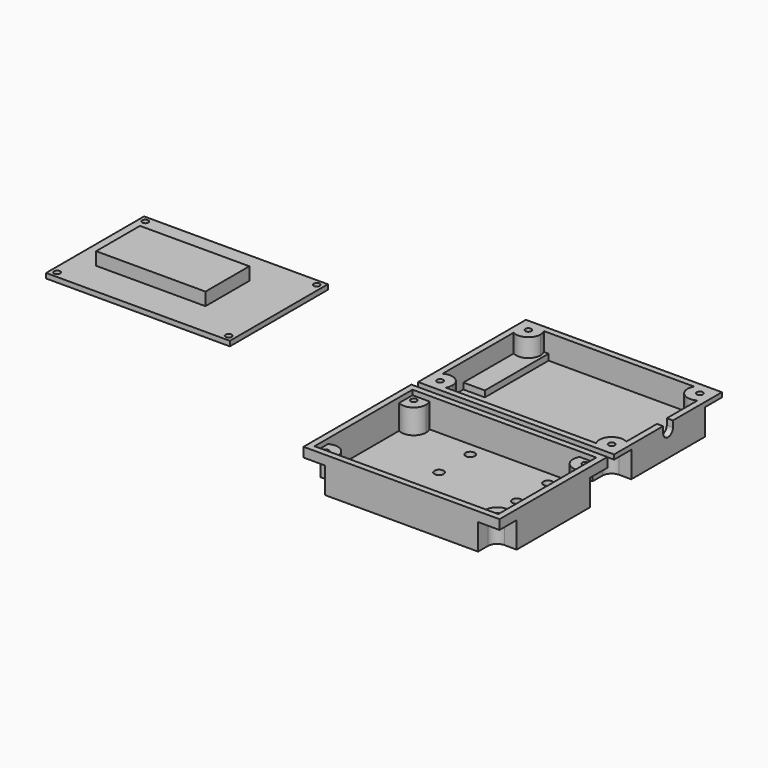
from build123d import *

# Parameters (mm, degrees)
F0_W      = 60
F0_H      = 40
F0_R      = 1
F1_DEPTH  = 1.6
F3_W      = 35.7
F3_H      = 17.9
F4_DEPTH  = 4.2
F5_W      = 64
F5_H      = 44
F5_R      = 1
F6_DEPTH  = 2
F7_R      = 1
F8_DEPTH  = 8
F9_W      = 64
F9_H      = 44
F9_R      = 1
F10_DEPTH = 2
F11_R     = 1
F12_DEPTH = 8
F13_W     = 64
F13_H     = 44
F13_W_2   = 60
F13_H_2   = 40
F14_DEPTH = 1.6
F16_DEPTH = 8.5
F18_DEPTH = 8.5
F20_DEPTH = 25.4
F21_R     = 1.5
F22_DEPTH = 25.4
F23_W     = 9
F23_H     = 28
F24_DEPTH = 4
F25_W     = 7
F25_H     = 26
F26_DEPTH = 2
F27_R     = 1
F28_DEPTH = 25.4


with BuildPart() as f1:
    # F0 (on Top) → F1 (new body)
    with BuildSketch(Plane.XY):
        with Locations((-71.7097583413, 11.8171558529)):
            Rectangle(F0_W, F0_H)
        with Locations((-99.7097583413, -6.1828441471)):
            Circle(F0_R, mode=Mode.SUBTRACT)
        with Locations((-43.7097583413, -6.1828441471)):
            Circle(F0_R, mode=Mode.SUBTRACT)
        with Locations((-99.7097583413, 29.8171558529)):
            Circle(F0_R, mode=Mode.SUBTRACT)
        with Locations((-43.7097583413, 29.8171558529)):
            Circle(F0_R, mode=Mode.SUBTRACT)
    extrude(amount=F1_DEPTH)

    # F3 (on face) → F4 (join)
    with BuildSketch(Plane.XY.offset(1.6)):
        with Locations((-76.3597583413, 11.8171558529)):
            Rectangle(F3_W, F3_H)
    extrude(amount=F4_DEPTH)


with BuildPart() as f6:
    # F5 (on Top) → F6 (new body)
    with BuildSketch(Plane.XY):
        with Locations((52.0504697859, 13.4392828941)):
            Rectangle(F5_W, F5_H)
        with Locations((24.0504697859, -4.5607171059)):
            Circle(F5_R, mode=Mode.SUBTRACT)
        with Locations((80.0504697859, -4.5607171059)):
            Circle(F5_R, mode=Mode.SUBTRACT)
        with Locations((24.0504697859, 31.4392828941)):
            Circle(F5_R, mode=Mode.SUBTRACT)
        with Locations((80.0504697859, 31.4392828941)):
            Circle(F5_R, mode=Mode.SUBTRACT)
    extrude(amount=F6_DEPTH)

    # F7 (on face) → F8 (join)
    with BuildSketch(Plane.XY.offset(2)):
        with BuildLine():
            Line((22.0504697859, 33.4392828941), (27.5145714011, 33.4392828941))
            ThreePointArc((27.5145714011, 33.4392828941), (26.0504697859, 34.9033845093), (24.0504697859, 35.4392828941))
            ThreePointArc((24.0504697859, 35.4392828941), (21.2220426612, 34.2677100189), (20.0504697859, 31.4392828941))
            ThreePointArc((20.0504697859, 31.4392828941), (20.5863681708, 29.4392828941), (22.0504697859, 27.975181279))
            Line((22.0504697859, 27.975181279), (22.0504697859, 33.4392828941))
        make_face()
        with BuildLine():
            ThreePointArc((24.0504697859, 35.4392828941), (26.0504697859, 34.9033845093), (27.5145714011, 33.4392828941))
            Line((27.5145714011, 33.4392828941), (76.5863681708, 33.4392828941))
            ThreePointArc((76.5863681708, 33.4392828941), (78.0504697859, 34.9033845093), (80.0504697859, 35.4392828941))
            Line((80.0504697859, 35.4392828941), (24.0504697859, 35.4392828941))
        make_face()
        with BuildLine():
            Line((22.0504697859, -1.0966154907), (22.0504697859, 27.975181279))
            ThreePointArc((22.0504697859, 27.975181279), (20.5863681708, 29.4392828941), (20.0504697859, 31.4392828941))
            Line((20.0504697859, 31.4392828941), (20.0504697859, -4.5607170954))
            ThreePointArc((20.0504697859, -4.5607170954), (20.5863681734, -2.5607171013), (22.0504697859, -1.0966154907))
        make_face()
        with BuildLine():
            ThreePointArc((20.0504697859, 31.4392828941), (21.2220426612, 34.2677100189), (24.0504697859, 35.4392828941))
            Line((24.0504697859, 35.4392828941), (20.0504697859, 35.4392828941))
            Line((20.0504697859, 35.4392828941), (20.0504697859, 31.4392828941))
        make_face()
        with BuildLine():
            ThreePointArc((80.0504697859, 35.4392828941), (78.0504697859, 34.9033845093), (76.5863681708, 33.4392828941))
            Line((76.5863681708, 33.4392828941), (82.0504697859, 33.4392828941))
            Line((82.0504697859, 33.4392828941), (82.0504697859, 27.975181279))
            ThreePointArc((82.0504697859, 27.975181279), (83.5145714011, 29.4392828941), (84.0504697859, 31.4392828941))
            ThreePointArc((84.0504697859, 31.4392828941), (82.8788969107, 34.2677100189), (80.0504697859, 35.4392828941))
        make_face()
        with BuildLine():
            Line((22.0504697859, -6.5607171059), (22.0504697859, -1.0966154907))
            ThreePointArc((22.0504697859, -1.0966154907), (20.5863681734, -2.5607171013), (20.0504697859, -4.5607170954))
            ThreePointArc((20.0504697859, -4.5607170954), (21.2220426575, -7.3891442269), (24.0504697859, -8.5607171059))
            ThreePointArc((24.0504697859, -8.5607171059), (26.0504697859, -8.024818721), (27.5145714011, -6.5607171059))
            Line((27.5145714011, -6.5607171059), (22.0504697859, -6.5607171059))
        make_face()
        with BuildLine():
            Line((84.0504697859, 35.4392828941), (80.0504697859, 35.4392828941))
            ThreePointArc((80.0504697859, 35.4392828941), (82.8788969107, 34.2677100189), (84.0504697859, 31.4392828941))
            Line((84.0504697859, 31.4392828941), (84.0504697859, 35.4392828941))
        make_face()
        with BuildLine():
            ThreePointArc((84.0504697859, 31.4392828941), (83.5145714011, 29.4392828941), (82.0504697859, 27.975181279))
            Line((82.0504697859, 27.975181279), (82.0504697859, -1.0966154907))
            ThreePointArc((82.0504697859, -1.0966154907), (83.5145714011, -2.5607171059), (84.0504697859, -4.5607171059))
            Line((84.0504697859, -4.5607171059), (84.0504697859, 31.4392828941))
        make_face()
        with BuildLine():
            ThreePointArc((24.0504697859, -8.5607171059), (21.2220426575, -7.3891442269), (20.0504697859, -4.5607170954))
            Line((20.0504697859, -4.5607170954), (20.0504697859, -8.5607171059))
            Line((20.0504697859, -8.5607171059), (24.0504697859, -8.5607171059))
        make_face()
        with BuildLine():
            ThreePointArc((84.0504697859, -4.5607171059), (83.5145714011, -2.5607171059), (82.0504697859, -1.0966154907))
            Line((82.0504697859, -1.0966154907), (82.0504697859, -6.5607171059))
            Line((82.0504697859, -6.5607171059), (76.5863681708, -6.5607171059))
            ThreePointArc((76.5863681708, -6.5607171059), (78.0504697859, -8.024818721), (80.0504697859, -8.5607171059))
            ThreePointArc((80.0504697859, -8.5607171059), (82.8788969107, -7.3891442306), (84.0504697859, -4.5607171059))
        make_face()
        with BuildLine():
            ThreePointArc((27.5145714011, -6.5607171059), (26.0504697859, -8.024818721), (24.0504697859, -8.5607171059))
            Line((24.0504697859, -8.5607171059), (80.0504697859, -8.5607171059))
            ThreePointArc((80.0504697859, -8.5607171059), (78.0504697859, -8.024818721), (76.5863681708, -6.5607171059))
            Line((76.5863681708, -6.5607171059), (27.5145714011, -6.5607171059))
        make_face()
        with BuildLine():
            Line((84.0504697859, -8.5607171059), (84.0504697859, -4.5607171059))
            ThreePointArc((84.0504697859, -4.5607171059), (82.8788969107, -7.3891442306), (80.0504697859, -8.5607171059))
            Line((80.0504697859, -8.5607171059), (84.0504697859, -8.5607171059))
        make_face()
        with BuildLine():
            ThreePointArc((22.0504697859, 27.975181279), (26.0504697859, 27.975181279), (28.0504697859, 31.4392828941))
            ThreePointArc((28.0504697859, 31.4392828941), (27.9141730911, 32.4745590745), (27.5145714011, 33.4392828941))
            Line((27.5145714011, 33.4392828941), (22.0504697859, 33.4392828941))
            Line((22.0504697859, 33.4392828941), (22.0504697859, 27.975181279))
        make_face()
        with Locations((24.0504697859, 31.4392828941)):
            Circle(F7_R, mode=Mode.SUBTRACT)
        with BuildLine():
            ThreePointArc((28.0504697859, -4.5607171059), (26.0504697859, -1.0966154907), (22.0504697859, -1.0966154907))
            Line((22.0504697859, -1.0966154907), (22.0504697859, -6.5607171059))
            Line((22.0504697859, -6.5607171059), (27.5145714011, -6.5607171059))
            ThreePointArc((27.5145714011, -6.5607171059), (27.9141730911, -5.5959932863), (28.0504697859, -4.5607171059))
        make_face()
        with Locations((24.0504697859, -4.5607171059)):
            Circle(F7_R, mode=Mode.SUBTRACT)
        with BuildLine():
            Line((82.0504697859, -6.5607171059), (82.0504697859, -1.0966154907))
            ThreePointArc((82.0504697859, -1.0966154907), (77.2220426612, -1.7322899811), (76.5863681708, -6.5607171059))
            Line((76.5863681708, -6.5607171059), (82.0504697859, -6.5607171059))
        make_face()
        with Locations((80.0504697859, -4.5607171059)):
            Circle(F7_R, mode=Mode.SUBTRACT)
        with BuildLine():
            Line((82.0504697859, 33.4392828941), (76.5863681708, 33.4392828941))
            ThreePointArc((76.5863681708, 33.4392828941), (77.2220426612, 28.6108557694), (82.0504697859, 27.975181279))
            Line((82.0504697859, 27.975181279), (82.0504697859, 33.4392828941))
        make_face()
        with Locations((80.0504697859, 31.4392828941)):
            Circle(F7_R, mode=Mode.SUBTRACT)
    extrude(amount=F8_DEPTH)

    # F17 (on face) → F18 (cut)
    with BuildSketch(Plane(origin=(0, 0, 0), x_dir=(1, 0, 0), z_dir=(0, 0, -1))):
        with BuildLine():
            ThreePointArc((80.0504697859, 1.5607171059), (82.1717901295, 2.4393967623), (83.0504697859, 4.5607171059))
            ThreePointArc((83.0504697859, 4.5607171059), (80.0504697859, 7.5607171059), (77.0504697859, 4.5607171059))
            ThreePointArc((77.0504697859, 4.5607171059), (77.9291494424, 2.4393967623), (80.0504697859, 1.5607171059))
        make_face()
        with BuildLine():
            ThreePointArc((77.0504697859, -31.4392828941), (80.0504697859, -34.4392828941), (83.0504697859, -31.4392828941))
            ThreePointArc((83.0504697859, -31.4392828941), (82.1717901295, -29.3179625506), (80.0504697859, -28.4392828941))
            ThreePointArc((80.0504697859, -28.4392828941), (77.9291494424, -29.3179625506), (77.0504697859, -31.4392828941))
        make_face()
        with BuildLine():
            ThreePointArc((24.0504697859, 1.5607171059), (26.1717901295, 2.4393967623), (27.0504697859, 4.5607171059))
            ThreePointArc((27.0504697859, 4.5607171059), (21.9291494424, 6.6820374494), (24.0504697859, 1.5607171059))
        make_face()
        with BuildLine():
            ThreePointArc((24.0504697859, -28.4392828941), (21.9291494424, -33.5606032377), (27.0504697859, -31.4392828941))
            ThreePointArc((27.0504697859, -31.4392828941), (26.1717901295, -29.3179625506), (24.0504697859, -28.4392828941))
        make_face()
        with BuildLine():
            ThreePointArc((77.0504697859, 4.5607171059), (80.0504697859, 7.5607171059), (83.0504697859, 4.5607171059))
            ThreePointArc((83.0504697859, 4.5607171059), (82.1717901295, 2.4393967623), (80.0504697859, 1.5607171059))
            Line((80.0504697859, 1.5607171059), (84.0504697859, 1.5607171059))
            Line((84.0504697859, 1.5607171059), (84.0504697859, 8.5607171059))
            Line((84.0504697859, 8.5607171059), (77.0504697859, 8.5607171059))
            Line((77.0504697859, 8.5607171059), (77.0504697859, 4.5607171059))
        make_face()
        with BuildLine():
            Line((84.0504697859, -35.4392828941), (84.0504697859, -28.4392828941))
            Line((84.0504697859, -28.4392828941), (80.0504697859, -28.4392828941))
            ThreePointArc((80.0504697859, -28.4392828941), (82.1717901295, -29.3179625506), (83.0504697859, -31.4392828941))
            ThreePointArc((83.0504697859, -31.4392828941), (80.0504697859, -34.4392828941), (77.0504697859, -31.4392828941))
            Line((77.0504697859, -31.4392828941), (77.0504697859, -35.4392828941))
            Line((77.0504697859, -35.4392828941), (84.0504697859, -35.4392828941))
        make_face()
        with BuildLine():
            Line((27.0504697859, 4.5607171059), (27.0504697859, 8.5607171059))
            Line((27.0504697859, 8.5607171059), (20.0504697859, 8.5607171059))
            Line((20.0504697859, 8.5607171059), (20.0504697859, 1.5607171059))
            Line((20.0504697859, 1.5607171059), (24.0504697859, 1.5607171059))
            ThreePointArc((24.0504697859, 1.5607171059), (21.9291494424, 6.6820374494), (27.0504697859, 4.5607171059))
        make_face()
        with BuildLine():
            Line((24.0504697859, -28.4392828941), (20.0504697859, -28.4392828941))
            Line((20.0504697859, -28.4392828941), (20.0504697859, -35.4392828941))
            Line((20.0504697859, -35.4392828941), (27.0504697859, -35.4392828941))
            Line((27.0504697859, -35.4392828941), (27.0504697859, -31.4392828941))
            ThreePointArc((27.0504697859, -31.4392828941), (21.9291494424, -33.5606032377), (24.0504697859, -28.4392828941))
        make_face()
    extrude(amount=-F18_DEPTH, mode=Mode.SUBTRACT)

    # F19 (on face) → F20 (cut)
    with BuildSketch(Plane.YZ.offset(84.0504697859)):
        with BuildLine():
            ThreePointArc((13.4392828941, 10), (12.0250693318, 9.4142135624), (11.4392828941, 8))
            ThreePointArc((11.4392828941, 8), (13.4392828941, 6), (15.4392828941, 8))
            ThreePointArc((15.4392828941, 8), (14.8534964565, 9.4142135624), (13.4392828941, 10))
        make_face()
        with BuildLine():
            ThreePointArc((13.4392828941, 10), (14.8534964565, 9.4142135624), (15.4392828941, 8))
            Line((15.4392828941, 8), (15.4392828941, 10))
            Line((15.4392828941, 10), (13.4392828941, 10))
        make_face()
        with BuildLine():
            Line((11.4392828941, 10), (11.4392828941, 8))
            ThreePointArc((11.4392828941, 8), (12.0250693318, 9.4142135624), (13.4392828941, 10))
            Line((13.4392828941, 10), (11.4392828941, 10))
        make_face()
    extrude(amount=-F20_DEPTH, mode=Mode.SUBTRACT)

    # F23 (on face) → F24 (join)
    with BuildSketch(Plane(origin=(0, 0, 0), x_dir=(1, 0, 0), z_dir=(0, 0, -1))):
        with Locations((24.5504697859, -21.4392828941)):
            Rectangle(F23_W, F23_H)
    extrude(amount=-F24_DEPTH)

    # F25 (on face) → F26 (cut)
    with BuildSketch(Plane(origin=(0, 0, 0), x_dir=(1, 0, 0), z_dir=(0, 0, -1))):
        with Locations((23.5504697859, -22.4392828941)):
            Rectangle(F25_W, F25_H)
    extrude(amount=-F26_DEPTH, mode=Mode.SUBTRACT)

    # F27 (on face) → F28 (cut)
    with BuildSketch(Plane(origin=(0, 0, 8.5), x_dir=(1, 0, 0), z_dir=(0, 0, -1))):
        with BuildLine():
            ThreePointArc((24.0504697859, -28.4392828941), (21.9291494424, -33.5606032377), (27.0504697859, -31.4392828941))
            ThreePointArc((27.0504697859, -31.4392828941), (26.1717901295, -29.3179625506), (24.0504697859, -28.4392828941))
        make_face()
        with Locations((24.0504697859, -31.4392828941)):
            Circle(F27_R, mode=Mode.SUBTRACT)
        with BuildLine():
            Line((20.0504697859, -28.4392828941), (20.0504697859, -35.4392828941))
            Line((20.0504697859, -35.4392828941), (27.0504697859, -35.4392828941))
            Line((27.0504697859, -35.4392828941), (27.0504697859, -31.4392828941))
            ThreePointArc((27.0504697859, -31.4392828941), (21.9291494424, -33.5606032377), (24.0504697859, -28.4392828941))
            Line((24.0504697859, -28.4392828941), (20.0504697859, -28.4392828941))
        make_face()
        with Locations((24.0504697859, -31.4392828941)):
            Circle(F27_R)
    extrude(amount=F28_DEPTH, mode=Mode.SUBTRACT)


with BuildPart() as f10:
    # F9 (on Top) → F10 (new body)
    with BuildSketch(Plane.XY):
        with Locations((53.5033790469, -35.1341663599)):
            Rectangle(F9_W, F9_H)
        with Locations((25.5033790469, -53.1341663599)):
            Circle(F9_R, mode=Mode.SUBTRACT)
        with Locations((81.5033790469, -53.1341663599)):
            Circle(F9_R, mode=Mode.SUBTRACT)
        with Locations((25.5033790469, -17.1341663599)):
            Circle(F9_R, mode=Mode.SUBTRACT)
        with Locations((81.5033790469, -17.1341663599)):
            Circle(F9_R, mode=Mode.SUBTRACT)
    extrude(amount=F10_DEPTH)

    # F11 (on face) → F12 (join)
    with BuildSketch(Plane.XY.offset(2)):
        with BuildLine():
            Line((23.5033790469, -15.1341663599), (28.9674806621, -15.1341663599))
            ThreePointArc((28.9674806621, -15.1341663599), (27.5033790469, -13.6700647448), (25.5033790469, -13.1341663599))
            ThreePointArc((25.5033790469, -13.1341663599), (22.6749519222, -14.3057392352), (21.5033790469, -17.1341663599))
            ThreePointArc((21.5033790469, -17.1341663599), (22.0392774318, -19.1341663599), (23.5033790469, -20.598267975))
            Line((23.5033790469, -20.598267975), (23.5033790469, -15.1341663599))
        make_face()
        with BuildLine():
            ThreePointArc((25.5033790469, -13.1341663599), (27.5033790469, -13.6700647448), (28.9674806621, -15.1341663599))
            Line((28.9674806621, -15.1341663599), (78.0392774318, -15.1341663599))
            ThreePointArc((78.0392774318, -15.1341663599), (79.5033790396, -13.670064749), (81.50337903, -13.1341663599))
            Line((81.50337903, -13.1341663599), (25.5033790469, -13.1341663599))
        make_face()
        with BuildLine():
            Line((23.5033790469, -49.6700647448), (23.5033790469, -20.598267975))
            ThreePointArc((23.5033790469, -20.598267975), (22.0392774318, -19.1341663599), (21.5033790469, -17.1341663599))
            Line((21.5033790469, -17.1341663599), (21.5033790469, -53.1341663599))
            ThreePointArc((21.5033790469, -53.1341663599), (22.0392774318, -51.1341663599), (23.5033790469, -49.6700647448))
        make_face()
        with BuildLine():
            ThreePointArc((21.5033790469, -17.1341663599), (22.6749519222, -14.3057392352), (25.5033790469, -13.1341663599))
            Line((25.5033790469, -13.1341663599), (21.5033790469, -13.1341663599))
            Line((21.5033790469, -13.1341663599), (21.5033790469, -17.1341663599))
        make_face()
        with BuildLine():
            ThreePointArc((81.50337903, -13.1341663599), (79.5033790396, -13.670064749), (78.0392774318, -15.1341663599))
            Line((78.0392774318, -15.1341663599), (83.5033790469, -15.1341663599))
            Line((83.5033790469, -15.1341663599), (83.5033790469, -20.598267975))
            ThreePointArc((83.5033790469, -20.598267975), (84.9674806621, -19.1341663599), (85.5033790469, -17.1341663599))
            ThreePointArc((85.5033790469, -17.1341663599), (84.3318061657, -14.3057392292), (81.50337903, -13.1341663599))
        make_face()
        with BuildLine():
            Line((23.5033790469, -55.1341663599), (23.5033790469, -49.6700647448))
            ThreePointArc((23.5033790469, -49.6700647448), (22.0392774318, -51.1341663599), (21.5033790469, -53.1341663599))
            ThreePointArc((21.5033790469, -53.1341663599), (22.6749519222, -55.9625934846), (25.5033790469, -57.1341663599))
            ThreePointArc((25.5033790469, -57.1341663599), (27.5033790469, -56.598267975), (28.9674806621, -55.1341663599))
            Line((28.9674806621, -55.1341663599), (23.5033790469, -55.1341663599))
        make_face()
        with BuildLine():
            Line((85.5033790469, -13.1341663599), (81.50337903, -13.1341663599))
            ThreePointArc((81.50337903, -13.1341663599), (84.3318061657, -14.3057392292), (85.5033790469, -17.1341663599))
            Line((85.5033790469, -17.1341663599), (85.5033790469, -13.1341663599))
        make_face()
        with BuildLine():
            ThreePointArc((85.5033790469, -17.1341663599), (84.9674806621, -19.1341663599), (83.5033790469, -20.598267975))
            Line((83.5033790469, -20.598267975), (83.5033790469, -49.6700647448))
            ThreePointArc((83.5033790469, -49.6700647448), (84.9674806621, -51.1341663599), (85.5033790469, -53.1341663599))
            Line((85.5033790469, -53.1341663599), (85.5033790469, -17.1341663599))
        make_face()
        with BuildLine():
            ThreePointArc((25.5033790469, -57.1341663599), (22.6749519222, -55.9625934846), (21.5033790469, -53.1341663599))
            Line((21.5033790469, -53.1341663599), (21.5033790469, -57.1341663599))
            Line((21.5033790469, -57.1341663599), (25.5033790469, -57.1341663599))
        make_face()
        with BuildLine():
            ThreePointArc((85.5033790469, -53.1341663599), (84.9674806621, -51.1341663599), (83.5033790469, -49.6700647448))
            Line((83.5033790469, -49.6700647448), (83.5033790469, -55.1341663599))
            Line((83.5033790469, -55.1341663599), (78.0392774318, -55.1341663599))
            ThreePointArc((78.0392774318, -55.1341663599), (79.5033790469, -56.598267975), (81.5033790469, -57.1341663599))
            ThreePointArc((81.5033790469, -57.1341663599), (84.3318061717, -55.9625934846), (85.5033790469, -53.1341663599))
        make_face()
        with BuildLine():
            ThreePointArc((28.9674806621, -55.1341663599), (27.5033790469, -56.598267975), (25.5033790469, -57.1341663599))
            Line((25.5033790469, -57.1341663599), (81.5033790469, -57.1341663599))
            ThreePointArc((81.5033790469, -57.1341663599), (79.5033790469, -56.598267975), (78.0392774318, -55.1341663599))
            Line((78.0392774318, -55.1341663599), (28.9674806621, -55.1341663599))
        make_face()
        with BuildLine():
            Line((85.5033790469, -57.1341663599), (85.5033790469, -53.1341663599))
            ThreePointArc((85.5033790469, -53.1341663599), (84.3318061717, -55.9625934846), (81.5033790469, -57.1341663599))
            Line((81.5033790469, -57.1341663599), (85.5033790469, -57.1341663599))
        make_face()
        with BuildLine():
            ThreePointArc((29.5033790469, -53.1341663599), (27.5033790469, -49.6700647448), (23.5033790469, -49.6700647448))
            Line((23.5033790469, -49.6700647448), (23.5033790469, -55.1341663599))
            Line((23.5033790469, -55.1341663599), (28.9674806621, -55.1341663599))
            ThreePointArc((28.9674806621, -55.1341663599), (29.3670823521, -54.1694425403), (29.5033790469, -53.1341663599))
        make_face()
        with Locations((25.5033790469, -53.1341663599)):
            Circle(F11_R, mode=Mode.SUBTRACT)
        with BuildLine():
            ThreePointArc((23.5033790469, -20.598267975), (27.5033790469, -20.598267975), (29.5033790469, -17.1341663599))
            ThreePointArc((29.5033790469, -17.1341663599), (29.3670823521, -16.0988901795), (28.9674806621, -15.1341663599))
            Line((28.9674806621, -15.1341663599), (23.5033790469, -15.1341663599))
            Line((23.5033790469, -15.1341663599), (23.5033790469, -20.598267975))
        make_face()
        with Locations((25.5033790469, -17.1341663599)):
            Circle(F11_R, mode=Mode.SUBTRACT)
        with BuildLine():
            Line((83.5033790469, -15.1341663599), (78.0392774318, -15.1341663599))
            ThreePointArc((78.0392774318, -15.1341663599), (78.6749519222, -19.9625934846), (83.5033790469, -20.598267975))
            Line((83.5033790469, -20.598267975), (83.5033790469, -15.1341663599))
        make_face()
        with Locations((81.5033790469, -17.1341663599)):
            Circle(F11_R, mode=Mode.SUBTRACT)
        with BuildLine():
            Line((83.5033790469, -55.1341663599), (83.5033790469, -49.6700647448))
            ThreePointArc((83.5033790469, -49.6700647448), (78.6749519222, -50.3057392352), (78.0392774318, -55.1341663599))
            Line((78.0392774318, -55.1341663599), (83.5033790469, -55.1341663599))
        make_face()
        with Locations((81.5033790469, -53.1341663599)):
            Circle(F11_R, mode=Mode.SUBTRACT)
    extrude(amount=F12_DEPTH)

    # F13 (on face) → F14 (join)
    with BuildSketch(Plane.XY.offset(10)):
        with Locations((53.5033790469, -35.1341663599)):
            Rectangle(F13_W, F13_H)
        with Locations((53.5033790469, -35.1341663599)):
            Rectangle(F13_W_2, F13_H_2, mode=Mode.SUBTRACT)
    extrude(amount=F14_DEPTH)

    # F15 (on face) → F16 (cut)
    with BuildSketch(Plane(origin=(0, 0, 0), x_dir=(1, 0, 0), z_dir=(0, 0, -1))):
        with BuildLine():
            ThreePointArc((81.5033790469, 50.1341663599), (83.6246993905, 51.0128460163), (84.5033790469, 53.1341663599))
            ThreePointArc((84.5033790469, 53.1341663599), (81.5033790469, 56.1341663599), (78.5033790469, 53.1341663599))
            ThreePointArc((78.5033790469, 53.1341663599), (79.3820587034, 51.0128460163), (81.5033790469, 50.1341663599))
        make_face()
        with BuildLine():
            ThreePointArc((78.5033790469, 17.1341663599), (81.5033790469, 14.1341663599), (84.5033790469, 17.1341663599))
            ThreePointArc((84.5033790469, 17.1341663599), (83.6246993905, 19.2554867035), (81.5033790469, 20.1341663599))
            ThreePointArc((81.5033790469, 20.1341663599), (79.3820587034, 19.2554867035), (78.5033790469, 17.1341663599))
        make_face()
        with BuildLine():
            ThreePointArc((25.5033790469, 50.1341663599), (27.6246993905, 51.0128460163), (28.5033790469, 53.1341663599))
            ThreePointArc((28.5033790469, 53.1341663599), (23.3820587034, 55.2554867035), (25.5033790469, 50.1341663599))
        make_face()
        with BuildLine():
            ThreePointArc((25.5033790469, 20.1341663599), (23.3820587034, 15.0128460163), (28.5033790469, 17.1341663599))
            ThreePointArc((28.5033790469, 17.1341663599), (27.6246993905, 19.2554867035), (25.5033790469, 20.1341663599))
        make_face()
        with BuildLine():
            Line((28.5033790469, 53.1341663599), (28.5033790469, 57.1341663599))
            Line((28.5033790469, 57.1341663599), (21.5033790469, 57.1341663599))
            Line((21.5033790469, 57.1341663599), (21.5033790469, 50.1341663599))
            Line((21.5033790469, 50.1341663599), (25.5033790469, 50.1341663599))
            ThreePointArc((25.5033790469, 50.1341663599), (23.3820587034, 55.2554867035), (28.5033790469, 53.1341663599))
        make_face()
        with BuildLine():
            Line((25.5033790469, 20.1341663599), (21.5033790469, 20.1341663599))
            Line((21.5033790469, 20.1341663599), (21.5033790469, 13.1341663599))
            Line((21.5033790469, 13.1341663599), (28.5033790469, 13.1341663599))
            Line((28.5033790469, 13.1341663599), (28.5033790469, 17.1341663599))
            ThreePointArc((28.5033790469, 17.1341663599), (23.3820587034, 15.0128460163), (25.5033790469, 20.1341663599))
        make_face()
        with BuildLine():
            Line((85.5033790469, 13.1341663599), (85.5033790469, 20.1341663599))
            Line((85.5033790469, 20.1341663599), (81.5033790469, 20.1341663599))
            ThreePointArc((81.5033790469, 20.1341663599), (83.6246993905, 19.2554867035), (84.5033790469, 17.1341663599))
            ThreePointArc((84.5033790469, 17.1341663599), (81.5033790469, 14.1341663599), (78.5033790469, 17.1341663599))
            Line((78.5033790469, 17.1341663599), (78.5033790469, 13.1341663599))
            Line((78.5033790469, 13.1341663599), (85.5033790469, 13.1341663599))
        make_face()
        with BuildLine():
            ThreePointArc((78.5033790469, 53.1341663599), (81.5033790469, 56.1341663599), (84.5033790469, 53.1341663599))
            ThreePointArc((84.5033790469, 53.1341663599), (83.6246993905, 51.0128460163), (81.5033790469, 50.1341663599))
            Line((81.5033790469, 50.1341663599), (85.5033790469, 50.1341663599))
            Line((85.5033790469, 50.1341663599), (85.5033790469, 57.1341663599))
            Line((85.5033790469, 57.1341663599), (78.5033790469, 57.1341663599))
            Line((78.5033790469, 57.1341663599), (78.5033790469, 53.1341663599))
        make_face()
    extrude(amount=-F16_DEPTH, mode=Mode.SUBTRACT)

    # F21 (on face) → F22 (cut)
    with BuildSketch(Plane(origin=(0, 0, 0), x_dir=(1, 0, 0), z_dir=(0, 0, -1))):
        with Locations((45.8033790469, 32.1841663599)):
            Circle(F21_R)
        with Locations((71.2033790469, 32.1841663599)):
            Circle(F21_R)
        with Locations((45.8033790469, 19.4841663599)):
            Circle(F21_R)
        with Locations((71.2033790469, 19.4841663599)):
            Circle(F21_R)
    extrude(amount=-F22_DEPTH, mode=Mode.SUBTRACT)


solid = Compound([f1.part, f6.part, f10.part])
